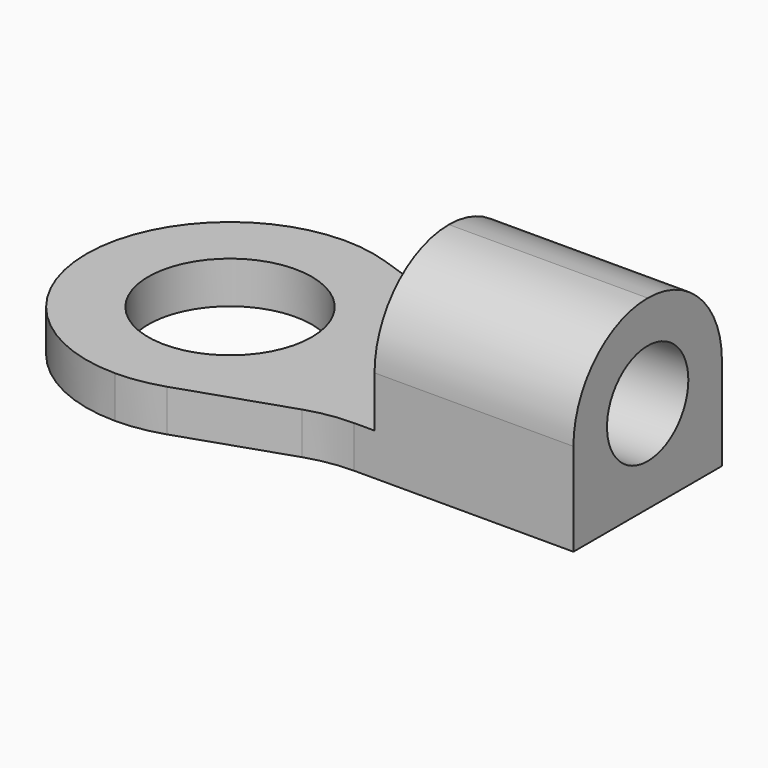
from build123d import *

# Parameters (mm, degrees)
F0_R     = 1.85
F1_DEPTH = 0.95
F2_W     = 4.5
F2_H     = 4.2
F3_DEPTH = 3.25
F4_R     = 2.09999
F5_R     = 1.15
F6_DEPTH = 25


# Not quite as in the source:
# - a fillet or chamfer is up to 0.001 mm smaller than in the source, because OpenCascade refuses the exact size


with BuildPart() as f1:
    # F0 (on Top) → F1 (new body)
    with BuildSketch(Plane.XY):
        with BuildLine():
            Line((8.2, 1.15), (12.7, 1.15))
            Line((12.7, 1.15), (12.7, 5.35))
            Line((12.7, 5.35), (8.2, 5.35))
            Line((8.2, 5.35), (7.7320977576, 5.35))
            ThreePointArc((7.7320977576, 5.35), (7.2069912058, 5.3927015871), (6.6956833513, 5.5196842405))
            Line((6.6956833513, 5.5196842405), (4.2864144063, 6.3303157595))
            ThreePointArc((4.2864144063, 6.3303157595), (3.7751065518, 6.4572984129), (3.25, 6.5))
            ThreePointArc((3.25, 6.5), (0.9519029611, 5.5480970389), (0, 3.25))
            ThreePointArc((0, 3.25), (0.9519029611, 0.9519029611), (3.25, 0))
            ThreePointArc((3.25, 0), (3.7751065518, 0.0427015871), (4.2864144063, 0.1696842405))
            Line((4.2864144063, 0.1696842405), (6.6956833513, 0.9803157595))
            ThreePointArc((6.6956833513, 0.9803157595), (7.2069912058, 1.1072984129), (7.7320977576, 1.15))
            Line((7.7320977576, 1.15), (8.2, 1.15))
        make_face()
        with Locations((3.25, 3.25)):
            Circle(F0_R, mode=Mode.SUBTRACT)
    extrude(amount=F1_DEPTH)

    # F2 (on face) → F3 (join)
    with BuildSketch(Plane.XY.offset(0.95)):
        with Locations((10.45, 3.25)):
            Rectangle(F2_W, F2_H)
    extrude(amount=F3_DEPTH)

    # F4 (radius 2.1 in the source; OpenCascade refuses exactly that, so slightly less here)
    f4_edges = [f1.edges().sort_by_distance(p)[0] for p in [
        (10.45, 5.35, 4.2),
        (10.45, 1.15, 4.2),
    ]]
    fillet(f4_edges, radius=F4_R)

    # F5 (on face) → F6 (cut)
    with BuildSketch(Plane.YZ.offset(12.7)):
        with Locations((3.25, 2.1)):
            Circle(F5_R)
    extrude(amount=-F6_DEPTH, mode=Mode.SUBTRACT)


solid = f1.part
